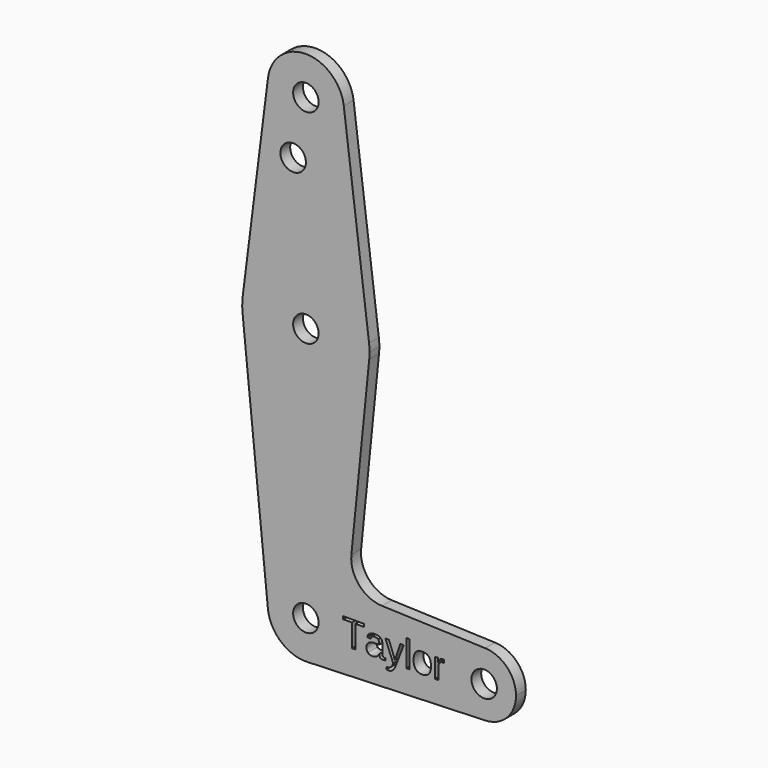
from build123d import *

# Parameters (mm, degrees)
F0_R     = 3.175
F0_W     = 0.8091993024
F0_H     = 6.6661924771
F1_DEPTH = 3.048


with BuildPart() as f1:
    # F0 (on Front) → F1 (new body)
    with BuildSketch(Plane.XZ):
        with BuildLine():
            ThreePointArc((44.7334821429, -7.9324362036), (50.1620069047, -5.5115227815), (52.3875, 0))
            ThreePointArc((52.3875, 0), (50.1620069047, 5.5115227815), (44.7334821429, 7.9324362036))
            ThreePointArc((44.7334821429, 7.9324362036), (36.5125, 0), (44.7334821429, -7.9324362036))
        make_face()
        with Locations((44.45, 0)):
            Circle(F0_R, mode=Mode.SUBTRACT)
        with BuildLine():
            ThreePointArc((44.7334821429, -7.9324362036), (36.5125, 0), (44.7334821429, 7.9324362036))
            Line((44.7334821429, 7.9324362036), (18.9676000005, 8.8532337108))
            ThreePointArc((18.9676000005, 8.8532337108), (13.2611998974, 11.5713591498), (11.3411865923, 17.5933818124))
            Line((11.3411865923, 17.5933818124), (15.7954255641, 61.9125))
            ThreePointArc((15.7954255641, 61.9125), (0, 47.625), (-15.7954255641, 61.9125))
            Line((-15.7954255641, 61.9125), (-9.4772553384, -0.9525))
            ThreePointArc((-9.4772553384, -0.9525), (-0.4768479324, 9.5130563464), (9.525, 0))
            ThreePointArc((9.525, 0), (6.8544082857, -6.6138273378), (0.3401785714, -9.5189234444))
            Line((0.3401785714, -9.5189234444), (44.7334821429, -7.9324362036))
        make_face()
        Polygon((14.4900061593, 2.7556789248), (12.3153728652, 2.7556789248), (12.3153728652, -2.8727837186), (11.4616172957, -2.8727837186), (11.4616172957, 2.7556789248), (9.2884213006, 2.7556789248), (9.2884213006, 3.4556435079), (14.4900061593, 3.4556435079), align=None, mode=Mode.SUBTRACT)
        with BuildLine():
            add(Edge.make_bspline(
                [(17.5586393932, -2.7319284226), (17.1475718967, -2.9633335517), (16.5597166308, -2.9633335517)],
                knots=[0, 0, 0, 1, 1, 1], degree=2))
            add(Edge.make_bspline(
                [(16.5597166308, -2.9633335517), (15.8266941722, -2.9633335517), (15.4587456439, -2.5767001373)],
                knots=[0, 0, 0, 1, 1, 1], degree=2))
            add(Edge.make_bspline(
                [(15.4587456439, -2.5767001373), (15.0907971156, -2.1900667228), (15.0907971156, -1.5159735206)],
                knots=[0, 0, 0, 1, 1, 1], degree=2))
            add(Edge.make_bspline(
                [(15.0907971156, -1.5159735206), (15.0907971156, -0.7613915778), (15.5873838989, -0.3575105761)],
                knots=[0, 0, 0, 1, 1, 1], degree=2))
            add(Edge.make_bspline(
                [(15.5873838989, -0.3575105761), (16.0839706822, 0.0463704256), (17.187816267, 0.0736791055)],
                knots=[0, 0, 0, 1, 1, 1], degree=2))
            Line((17.187816267, 0.0736791055), (18.2801634603, 0.0923639917))
            Line((18.2801634603, 0.0923639917), (18.2801634603, 0.3568269964))
            add(Edge.make_bspline(
                [(18.2801634603, 0.3568269964), (18.2801634603, 0.9489941591), (18.0286361461, 1.2055520196)],
                knots=[0, 0, 0, 1, 1, 1], degree=2))
            add(Edge.make_bspline(
                [(18.0286361461, 1.2055520196), (17.7771088318, 1.4621098801), (17.2381217298, 1.4621098801)],
                knots=[0, 0, 0, 1, 1, 1], degree=2))
            add(Edge.make_bspline(
                [(17.2381217298, 1.4621098801), (16.6948227311, 1.4621098801), (16.4476073136, 1.2774169665)],
                knots=[0, 0, 0, 1, 1, 1], degree=2))
            add(Edge.make_bspline(
                [(16.4476073136, 1.2774169665), (16.2003918962, 1.0927240529), (16.1500864334, 0.6888430512)],
                knots=[0, 0, 0, 1, 1, 1], degree=2))
            Line((16.1500864334, 0.6888430512), (15.3063919564, 0.7650198949))
            add(Edge.make_bspline(
                [(15.3063919564, 0.7650198949), (15.5133630036, 2.0772738258), (17.2553693171, 2.0772738258)],
                knots=[0, 0, 0, 1, 1, 1], degree=2))
            add(Edge.make_bspline(
                [(17.2553693171, 2.0772738258), (18.1723660399, 2.0772738258), (18.6344576487, 1.6568638863)],
                knots=[0, 0, 0, 1, 1, 1], degree=2))
            add(Edge.make_bspline(
                [(18.6344576487, 1.6568638863), (19.0965492574, 1.2364539468), (19.0965492574, 0.4416276337)],
                knots=[0, 0, 0, 1, 1, 1], degree=2))
            Line((19.0965492574, 0.4416276337), (19.0965492574, -1.6510796208))
            add(Edge.make_bspline(
                [(19.0965492574, -1.6510796208), (19.0965492574, -2.0104043555), (19.1914109874, -2.1922226712)],
                knots=[0, 0, 0, 1, 1, 1], degree=2))
            add(Edge.make_bspline(
                [(19.1914109874, -2.1922226712), (19.2862727173, -2.3740409869), (19.550735722, -2.3740409869)],
                knots=[0, 0, 0, 1, 1, 1], degree=2))
            add(Edge.make_bspline(
                [(19.550735722, -2.3740409869), (19.667156936, -2.3740409869), (19.8151987267, -2.3424204103)],
                knots=[0, 0, 0, 1, 1, 1], degree=2))
            Line((19.8151987267, -2.3424204103), (19.8151987267, -2.8454750388))
            add(Edge.make_bspline(
                [(19.8151987267, -2.8454750388), (19.5104913517, -2.9173399857), (19.1914109874, -2.9173399857)],
                knots=[0, 0, 0, 1, 1, 1], degree=2))
            add(Edge.make_bspline(
                [(19.1914109874, -2.9173399857), (18.7429737185, -2.9173399857), (18.5381586198, -2.6816229598)],
                knots=[0, 0, 0, 1, 1, 1], degree=2))
            add(Edge.make_bspline(
                [(18.5381586198, -2.6816229598), (18.333343521, -2.4459059338), (18.3060348412, -1.9428513053)],
                knots=[0, 0, 0, 1, 1, 1], degree=2))
            Line((18.3060348412, -1.9428513053), (18.2801634603, -1.9428513053))
            add(Edge.make_bspline(
                [(18.2801634603, -1.9428513053), (17.9697068896, -2.5005232935), (17.5586393932, -2.7319284226)],
                knots=[0, 0, 0, 1, 1, 1], degree=2))
        make_face(mode=Mode.SUBTRACT)
        with BuildLine():
            add(Edge.make_bspline(
                [(21.3897597139, -4.5953864965), (21.072835298, -4.781516709), (20.673266193, -4.781516709)],
                knots=[0, 0, 0, 1, 1, 1], degree=2))
            add(Edge.make_bspline(
                [(20.673266193, -4.781516709), (20.3412501382, -4.781516709), (20.1155942049, -4.7326485451)],
                knots=[0, 0, 0, 1, 1, 1], degree=2))
            Line((20.1155942049, -4.7326485451), (20.1155942049, -4.126108393))
            add(Edge.make_bspline(
                [(20.1155942049, -4.126108393), (20.2866327786, -4.1534170729), (20.4936038257, -4.1534170729)],
                knots=[0, 0, 0, 1, 1, 1], degree=2))
            add(Edge.make_bspline(
                [(20.4936038257, -4.1534170729), (21.2481857685, -4.1534170729), (21.6879992437, -3.0438222923)],
                knots=[0, 0, 0, 1, 1, 1], degree=2))
            Line((21.6879992437, -3.0438222923), (21.7641760874, -2.8497869356))
            Line((21.7641760874, -2.8497869356), (19.8381955097, 1.9867239927))
            Line((19.8381955097, 1.9867239927), (20.7005748729, 1.9867239927))
            Line((20.7005748729, 1.9867239927), (21.7239317171, -0.6981504245))
            add(Edge.make_bspline(
                [(21.7239317171, -0.6981504245), (21.7469285001, -0.7613915778), (21.7785490768, -0.8490668131)],
                knots=[0, 0, 0, 1, 1, 1], degree=2))
            add(Edge.make_bspline(
                [(21.7785490768, -0.8490668131), (21.8101696534, -0.9367420483), (21.9804895777, -1.43548478)],
                knots=[0, 0, 0, 1, 1, 1], degree=2))
            add(Edge.make_bspline(
                [(21.9804895777, -1.43548478), (22.1508095019, -1.9342275117), (22.1637451923, -1.9917194693)],
                knots=[0, 0, 0, 1, 1, 1], degree=2))
            Line((22.1637451923, -1.9917194693), (22.4785136599, -1.107780622))
            Line((22.4785136599, -1.107780622), (23.5435521734, 1.9867239927))
            Line((23.5435521734, 1.9867239927), (24.3973077429, 1.9867239927))
            Line((24.3973077429, 1.9867239927), (22.5288191227, -2.8727837186))
            add(Edge.make_bspline(
                [(22.5288191227, -2.8727837186), (22.2269863456, -3.6503624444), (21.9668352377, -4.0298093641)],
                knots=[0, 0, 0, 1, 1, 1], degree=2))
            add(Edge.make_bspline(
                [(21.9668352377, -4.0298093641), (21.7066841299, -4.4092562839), (21.3897597139, -4.5953864965)],
                knots=[0, 0, 0, 1, 1, 1], degree=2))
        make_face(mode=Mode.SUBTRACT)
        with Locations((25.4386308239, 0.4603125199)):
            Rectangle(F0_W, F0_H, mode=Mode.SUBTRACT)
        with BuildLine():
            add(Edge.make_bspline(
                [(30.6624938161, 1.4642658285), (31.1885452276, 0.8512578312), (31.1885452276, -0.4379993167)],
                knots=[0, 0, 0, 1, 1, 1], degree=2))
            add(Edge.make_bspline(
                [(31.1885452276, -0.4379993167), (31.1885452276, -1.7143207741), (30.6265613426, -2.3388271629)],
                knots=[0, 0, 0, 1, 1, 1], degree=2))
            add(Edge.make_bspline(
                [(30.6265613426, -2.3388271629), (30.0645774576, -2.9633335517), (28.9966643463, -2.9633335517)],
                knots=[0, 0, 0, 1, 1, 1], degree=2))
            add(Edge.make_bspline(
                [(28.9966643463, -2.9633335517), (27.9316258328, -2.9633335517), (27.388326834, -2.3136744315)],
                knots=[0, 0, 0, 1, 1, 1], degree=2))
            add(Edge.make_bspline(
                [(27.388326834, -2.3136744315), (26.8450278353, -1.6640153113), (26.8450278353, -0.4379993167)],
                knots=[0, 0, 0, 1, 1, 1], degree=2))
            add(Edge.make_bspline(
                [(26.8450278353, -0.4379993167), (26.8450278353, 2.0772738258), (29.0225357272, 2.0772738258)],
                knots=[0, 0, 0, 1, 1, 1], degree=2))
            add(Edge.make_bspline(
                [(29.0225357272, 2.0772738258), (30.1364424046, 2.0772738258), (30.6624938161, 1.4642658285)],
                knots=[0, 0, 0, 1, 1, 1], degree=2))
        make_face(mode=Mode.SUBTRACT)
        with BuildLine():
            Line((33.0196640753, -2.8727837186), (32.2119020719, -2.8727837186))
            Line((32.2119020719, -2.8727837186), (32.2119020719, 0.8555697281))
            add(Edge.make_bspline(
                [(32.2119020719, 0.8555697281), (32.2119020719, 1.3672481502), (32.184593392, 1.9867239927)],
                knots=[0, 0, 0, 1, 1, 1], degree=2))
            Line((32.184593392, 1.9867239927), (32.9477991284, 1.9867239927))
            add(Edge.make_bspline(
                [(32.9477991284, 1.9867239927), (32.9837316019, 1.160277103), (32.9837316019, 0.9949877251)],
                knots=[0, 0, 0, 1, 1, 1], degree=2))
            Line((32.9837316019, 0.9949877251), (33.0024164881, 0.9949877251))
            add(Edge.make_bspline(
                [(33.0024164881, 0.9949877251), (33.1950145459, 1.6187754644), (33.4465418601, 1.8480246451)],
                knots=[0, 0, 0, 1, 1, 1], degree=2))
            add(Edge.make_bspline(
                [(33.4465418601, 1.8480246451), (33.6980691744, 2.0772738258), (34.1565675358, 2.0772738258)],
                knots=[0, 0, 0, 1, 1, 1], degree=2))
            add(Edge.make_bspline(
                [(34.1565675358, 2.0772738258), (34.3175450169, 2.0772738258), (34.4842716938, 2.0327175587)],
                knots=[0, 0, 0, 1, 1, 1], degree=2))
            Line((34.4842716938, 2.0327175587), (34.4842716938, 1.2910713064))
            add(Edge.make_bspline(
                [(34.4842716938, 1.2910713064), (34.3232942126, 1.3356275735), (34.0530820122, 1.3356275735)],
                knots=[0, 0, 0, 1, 1, 1], degree=2))
            add(Edge.make_bspline(
                [(34.0530820122, 1.3356275735), (33.5500273837, 1.3356275735), (33.2848457295, 0.9022819436)],
                knots=[0, 0, 0, 1, 1, 1], degree=2))
            add(Edge.make_bspline(
                [(33.2848457295, 0.9022819436), (33.0196640753, 0.4689363136), (33.0196640753, -0.3388256899)],
                knots=[0, 0, 0, 1, 1, 1], degree=2))
            Line((33.0196640753, -0.3388256899), (33.0196640753, -2.8727837186))
        make_face(mode=Mode.SUBTRACT)
        with BuildLine():
            ThreePointArc((-9.4772553384, -0.9525), (-6.2623833816, -7.1769199091), (0.3401785714, -9.5189234444))
            ThreePointArc((0.3401785714, -9.5189234444), (6.8544082857, -6.6138273378), (9.525, 0))
            ThreePointArc((9.525, 0), (-0.4768479324, 9.5130563464), (-9.4772553384, -0.9525))
        make_face()
        Circle(F0_R, mode=Mode.SUBTRACT)
        with BuildLine():
            ThreePointArc((-15.7954255641, 61.9125), (0, 47.625), (15.7954255641, 61.9125))
            ThreePointArc((15.7954255641, 61.9125), (15.8550939106, 62.7052534459), (15.875, 63.5))
            ThreePointArc((15.875, 63.5), (15.8438414904, 64.4941387366), (15.7504882737, 65.484375))
            ThreePointArc((15.7504882737, 65.484375), (0, 79.375), (-15.7504882737, 65.484375))
            ThreePointArc((-15.7504882737, 65.484375), (-15.8737438155, 63.6997054867), (-15.7954255641, 61.9125))
        make_face()
        with Locations((0, 63.5)):
            Circle(F0_R, mode=Mode.SUBTRACT)
        with BuildLine():
            Line((-9.4502929642, 115.490625), (-15.7504882737, 65.484375))
            ThreePointArc((-15.7504882737, 65.484375), (0, 79.375), (15.7504882737, 65.484375))
            Line((15.7504882737, 65.484375), (9.4502929642, 115.490625))
            ThreePointArc((9.4502929642, 115.490625), (9.5063048942, 114.896483242), (9.525, 114.3))
            ThreePointArc((9.525, 114.3), (-0.596483242, 104.7936951058), (-9.4502929642, 115.490625))
        make_face()
        with Locations((-3.175, 100.0252)):
            Circle(F0_R, mode=Mode.SUBTRACT)
        with BuildLine():
            ThreePointArc((9.4502929642, 115.490625), (0, 123.825), (-9.4502929642, 115.490625))
            ThreePointArc((-9.4502929642, 115.490625), (-0.596483242, 104.7936951058), (9.525, 114.3))
            ThreePointArc((9.525, 114.3), (9.5063048942, 114.896483242), (9.4502929642, 115.490625))
        make_face()
        with Locations((0, 114.3)):
            Circle(F0_R, mode=Mode.SUBTRACT)
    extrude(amount=F1_DEPTH)


solid = f1.part
